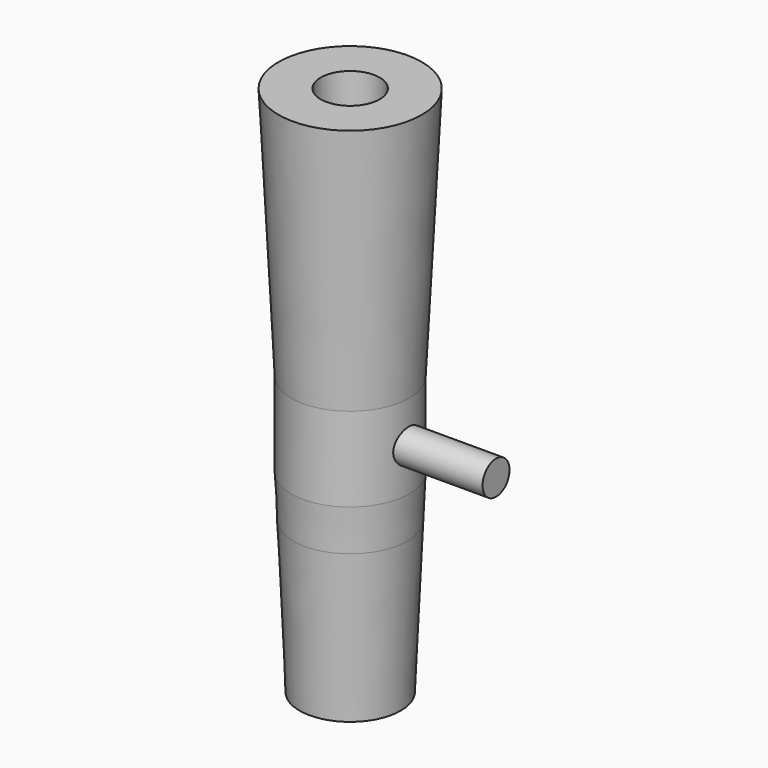
from build123d import *

# Parameters (mm, degrees)
F3_R     = 2
F4_DEPTH = 12.6554723829


with BuildPart() as f1:
    # F0 (on Front) → F1 (revolve)
    with BuildSketch(Plane.XZ):
        Polygon((2.5, 0), (1.5, 0), (1.5, -5), (4.7805098866, -5), (6.7824029301, -5), (7, 0), align=None)
        Polygon((2.6259404258, 5.0502821417), (2.5, 0), (7, 0), (7, 5.0502821417), (4.8129702129, 5.0502821417), align=None)
        Polygon((2.7508953229, 10.0610440238), (2.6259404258, 5.0502821417), (4.8129702129, 5.0502821417), (7, 5.0502821417), (7, 10), align=None)
        Polygon((4.7805098866, -5), (3.9981069565, -22.9782505862), (6, -22.9782505862), (6.7824029301, -5), align=None)
        Polygon((3.5, 40.1005642833), (2.7508953229, 10.0610440238), (7, 10), (8.5, 40.1005642833), align=None)
    revolve(axis=Axis((0, 0, 25.1005642833), (0, 0, 1)))

    # F3 (on line) → F4 (join)
    with BuildSketch(Plane.YZ.offset(17.3129702129)):
        with Locations((0, 5.0502821417)):
            Circle(F3_R)
    extrude(amount=-F4_DEPTH)


solid = f1.part
